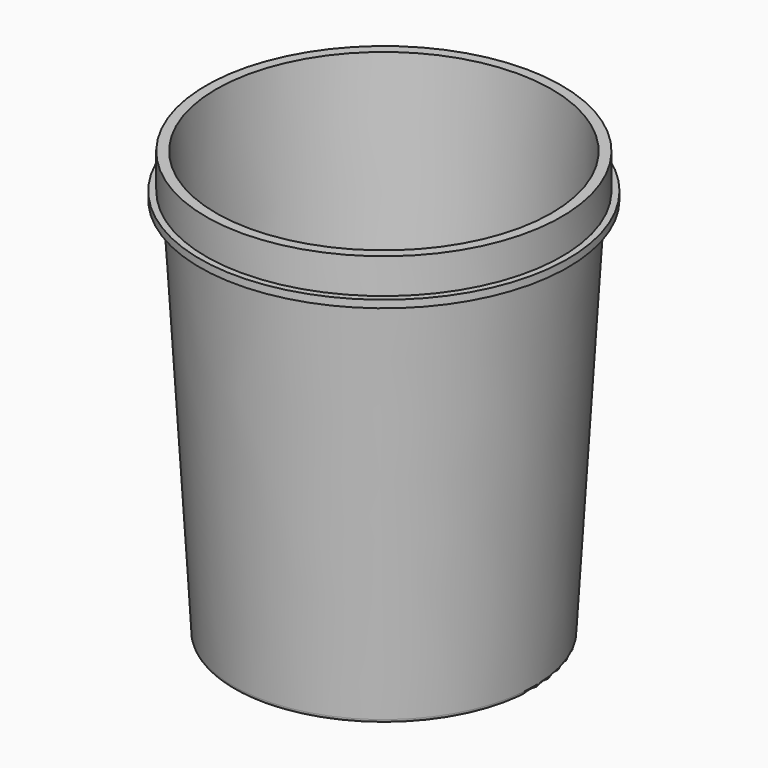
from build123d import *

# Parameters (mm, degrees)
F2_R = 1.49999


# Not quite as in the source:
# - a fillet or chamfer is up to 0.001 mm smaller than in the source, because OpenCascade refuses the exact size


with BuildPart() as f1:
    # F0 (on Right) → F1 (revolve)
    with BuildSketch(Plane.YZ):
        Polygon((43, 3), (43, 0), (60, 0), (69.0046720892, 153), (73.5, 153), (73.5, 156), (71, 156), (71, 170), (67, 170), (57.1713709877, 3), (46, 3), (46, 6), (0, 6), (0, 3), align=None)
    revolve(axis=Axis((0, 0, 4.5), (0, 0, -1)))

    # F2 (radius 1.5 in the source; OpenCascade refuses exactly that, so slightly less here)
    f2_edges = [f1.edges().sort_by_distance(p)[0] for p in [
        (0, -43, 0),
        (0, -60, 0),
        (0, -43, 3),
    ]]
    fillet(f2_edges, radius=F2_R)


solid = f1.part
